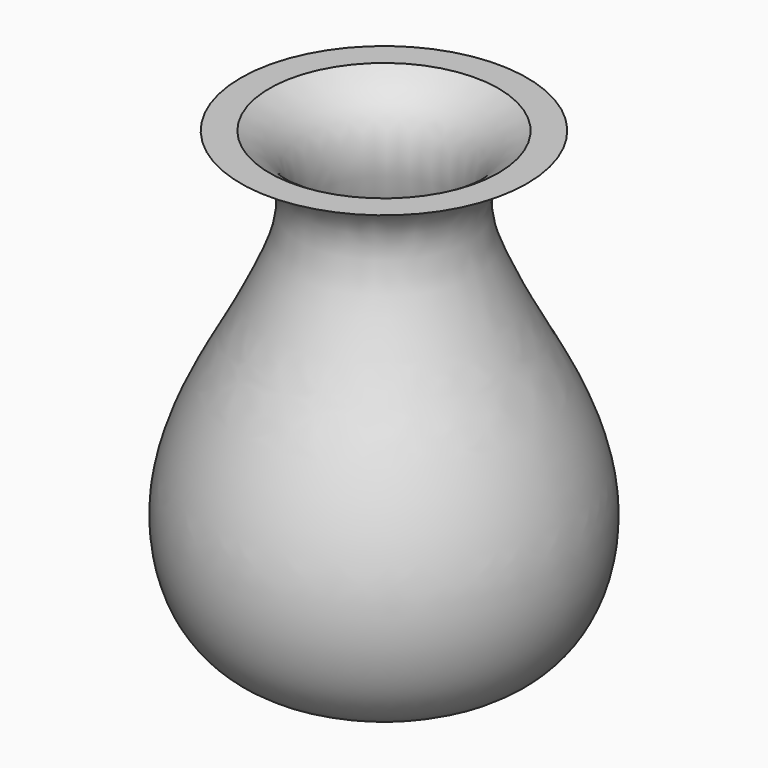
from build123d import *

# Parameters (mm, degrees)
F3_R     = 9.4302496374
F4_DEPTH = 6


# Not quite as in the source:
# - ends of sketch curves that miss each other by under 0.0002 mm in the source are joined
# - the dataset's text gives a spline's control points without its knots; the knots are read off the source's solid


with BuildPart() as f1:
    # F0 (on Front) → F1 (revolve)
    with BuildSketch(Plane.XZ):
        with BuildLine():
            add(Edge.make_bspline(
                [(30, 75.2996280789), (12.0761917662, 69.9585662546), (22.0660075591, 46.676498365), (27.6966733214, 36.2218981282), (42.7063983627, 9.1057052867), (34.5811633648, -19.2495821704), (17.7899881188, -23.4487943823), (14.7886006228, -24.1117397402)],
                knots=[0, 0, 0, 0, 0.1815872534, 0.3121168672, 0.4958376177, 0.6870531162, 0.7613433038, 0.7613433038, 0.7613433038, 0.7613433038], degree=3))
            Line((30, 75.2996280789), (23.9999937812, 75.2996280789))
            add(Edge.make_bspline(
                [(23.9999937812, 75.2996280789), (23.0401652673, 74.7936187135), (21.0247588483, 73.5335074467), (18.5585291762, 71.2374375612), (16.7198379267, 68.4175594433), (15.6826696477, 65.4130506141), (15.331612914, 62.3713239622), (15.5126860744, 59.3815893599), (16.0825011592, 56.4910760238), (16.916705774, 53.735455434), (17.7387201772, 51.5831610633), (18.4189479706, 49.9704141376), (18.9272543321, 48.8216741349), (19.4200549077, 47.7419083495), (20.0398236053, 46.399710855), (20.761807686, 44.8611954438), (21.562965975, 43.197405411), (22.321250427, 41.6663703234), (23.3029927321, 39.7404596384), (24.2824625412, 37.8948692714), (25.343200206, 35.9421986679), (26.2036248268, 34.371647892), (27.1429247952, 32.659191045), (28.4652186968, 30.2061159952), (30.1973374203, 26.8366561034), (32.2218636423, 22.3857513618), (34.0118488472, 17.6106526585), (35.1592588041, 13.4348404718), (35.785448931, 10.0199360293), (36.1877986343, 6.5714727134), (36.2397252491, 2.1938313072), (35.5493802078, -2.9499350247), (34.0820339451, -7.7778609851), (32.2029522741, -11.3746917966), (30.3010280758, -13.9131417929), (28.6716145167, -15.6306743639), (27.1396783972, -16.8932037461), (25.803572558, -17.7950920184), (24.39420105, -18.619315045), (22.4500071463, -19.5323385504), (20.4021028111, -20.2844311556), (18.7807315029, -20.7948544502), (17.592772776, -21.134210518), (16.452031039, -21.4325127884), (15.3771894816, -21.6925038619), (14.5514142739, -21.8797412312), (13.9410981585, -22.0135668432), (13.5103701444, -22.1064333576), (13.1083048799, -22.192326543), (12.7361659904, -22.2718756926), (12.3945880535, -22.3458779112), (12.0829949511, -22.4154919187), (11.8460619557, -22.4713734196), (11.6659844883, -22.5167836099), (11.5334752407, -22.5521765476), (11.4001289551, -22.5904987487), (11.2601656039, -22.6346104606), (11.1030535346, -22.6906076905), (10.9416605144, -22.7575957417), (10.7728572344, -22.8425122924), (10.6167334994, -22.9333364829), (10.4180576805, -23.0719896525), (10.1623729849, -23.2989454947), (9.8981203684, -23.6304309896), (9.7130739302, -24.0099991802), (9.6451369281, -24.2229738932), (9.6219207987, -24.3173828521)],
                knots=[0.0193804615, 0.0193804615, 0.0193804615, 0.0193804615, 0.0313625372, 0.0470438057, 0.0627250743, 0.0784063429, 0.0940876115, 0.1097688801, 0.1254501486, 0.1411314172, 0.1568126858, 0.1646533201, 0.1724939544, 0.1803345887, 0.188175223, 0.2038564915, 0.2195377601, 0.2352190287, 0.2509002973, 0.2822628344, 0.297944103, 0.3136253716, 0.3293066402, 0.3449879088, 0.3763504459, 0.4077129831, 0.4390755202, 0.4704380574, 0.486119326, 0.5018005946, 0.5331631317, 0.5645256689, 0.595888206, 0.6272507432, 0.6429320118, 0.6586132804, 0.6742945489, 0.6821351832, 0.6899758175, 0.7056570861, 0.7213383547, 0.729178989, 0.7370196233, 0.7448602576, 0.7527008918, 0.7605415261, 0.7644618433, 0.7683821604, 0.7723024776, 0.7762227947, 0.7801431119, 0.784063429, 0.7879837462, 0.7899439047, 0.7919040633, 0.7938642219, 0.7958243804, 0.797784539, 0.7997446976, 0.8007247769, 0.8017048562, 0.8026849354, 0.8036650147, 0.804645094, 0.8051351337, 0.8054861615, 0.8054861615, 0.8054861615, 0.8054861615], degree=3))
            Line((9.6219207987, -24.3173828521), (14.7886006228, -24.1117397402))
        make_face()
    revolve(axis=Axis((0, 0, 25.2996280789), (0, 0, -1)))


with BuildPart() as f1b:
    # F0 (on Front) → F1, piece 2 (revolve)
    with BuildSketch(Plane.XZ):
        with BuildLine():
            add(Edge.make_bspline(
                [(23.9999937812, 75.2996399804), (23.0401652673, 74.7936187135), (21.0247588483, 73.5335074467), (18.5585291762, 71.2374375612), (16.7198379267, 68.4175594433), (15.6826696477, 65.4130506141), (15.331612914, 62.3713239622), (15.5126860744, 59.3815893599), (16.0825011592, 56.4910760238), (16.916705774, 53.735455434), (17.7387201772, 51.5831610633), (18.4189479706, 49.9704141376), (18.9272543321, 48.8216741349), (19.4200549077, 47.7419083495), (20.0398236053, 46.399710855), (20.761807686, 44.8611954438), (21.562965975, 43.197405411), (22.321250427, 41.6663703234), (23.3029927321, 39.7404596384), (24.2824625412, 37.8948692714), (25.343200206, 35.9421986679), (26.2036248268, 34.371647892), (27.1429247952, 32.659191045), (28.4652186968, 30.2061159952), (30.1973374203, 26.8366561034), (32.2218636423, 22.3857513618), (34.0118488472, 17.6106526585), (35.1592588041, 13.4348404718), (35.785448931, 10.0199360293), (36.1877986343, 6.5714727134), (36.2397252491, 2.1938313072), (35.5493802078, -2.9499350247), (34.0820339451, -7.7778609851), (32.2029522741, -11.3746917966), (30.3010280758, -13.9131417929), (28.6716145167, -15.6306743639), (27.1396783972, -16.8932037461), (25.803572558, -17.7950920184), (24.39420105, -18.619315045), (22.4500071463, -19.5323385504), (20.4021028111, -20.2844311556), (18.7807315029, -20.7948544502), (17.592772776, -21.134210518), (16.452031039, -21.4325127884), (15.3771894816, -21.6925038619), (14.5514142739, -21.8797412312), (13.9410981585, -22.0135668432), (13.5103701444, -22.1064333576), (13.1083048799, -22.192326543), (12.7361659904, -22.2718756926), (12.3945880535, -22.3458779112), (12.0829949511, -22.4154919187), (11.8460619557, -22.4713734196), (11.6659844883, -22.5167836099), (11.5334752407, -22.5521765476), (11.4001289551, -22.5904987487), (11.2601656039, -22.6346104606), (11.1030535346, -22.6906076905), (10.9416605144, -22.7575957417), (10.7728572344, -22.8425122924), (10.6167334994, -22.9333364829), (10.4180576805, -23.0719896525), (10.1623729849, -23.2989454947), (9.8981203684, -23.6304309896), (9.7130739302, -24.0099991802), (9.6451369281, -24.2229738932), (9.6219207987, -24.3173828521)],
                knots=[0.0193804615, 0.0193804615, 0.0193804615, 0.0193804615, 0.0313625372, 0.0470438057, 0.0627250743, 0.0784063429, 0.0940876115, 0.1097688801, 0.1254501486, 0.1411314172, 0.1568126858, 0.1646533201, 0.1724939544, 0.1803345887, 0.188175223, 0.2038564915, 0.2195377601, 0.2352190287, 0.2509002973, 0.2822628344, 0.297944103, 0.3136253716, 0.3293066402, 0.3449879088, 0.3763504459, 0.4077129831, 0.4390755202, 0.4704380574, 0.486119326, 0.5018005946, 0.5331631317, 0.5645256689, 0.595888206, 0.6272507432, 0.6429320118, 0.6586132804, 0.6742945489, 0.6821351832, 0.6899758175, 0.7056570861, 0.7213383547, 0.729178989, 0.7370196233, 0.7448602576, 0.7527008918, 0.7605415261, 0.7644618433, 0.7683821604, 0.7723024776, 0.7762227947, 0.7801431119, 0.784063429, 0.7879837462, 0.7899439047, 0.7919040633, 0.7938642219, 0.7958243804, 0.797784539, 0.7997446976, 0.8007247769, 0.8017048562, 0.8026849354, 0.8036650147, 0.804645094, 0.8051351337, 0.8054861615, 0.8054861615, 0.8054861615, 0.8054861615], degree=3))
            Line((23.9999937812, 75.2996399804), (0, 75.2996280789))
            Line((0, 75.2996280789), (0, -24.7003719211))
            Line((0, -24.7003719211), (9.6219207987, -24.3173828521))
        make_face()
    revolve(axis=Axis((0, 0, 25.2996280789), (0, 0, -1)))

    # F0 (on Front) → F2 (revolve, cut)
    with BuildSketch(Plane.XZ):
        with BuildLine():
            add(Edge.make_bspline(
                [(23.9999937812, 75.2996399804), (23.0401652673, 74.7936187135), (21.0247588483, 73.5335074467), (18.5585291762, 71.2374375612), (16.7198379267, 68.4175594433), (15.6826696477, 65.4130506141), (15.331612914, 62.3713239622), (15.5126860744, 59.3815893599), (16.0825011592, 56.4910760238), (16.916705774, 53.735455434), (17.7387201772, 51.5831610633), (18.4189479706, 49.9704141376), (18.9272543321, 48.8216741349), (19.4200549077, 47.7419083495), (20.0398236053, 46.399710855), (20.761807686, 44.8611954438), (21.562965975, 43.197405411), (22.321250427, 41.6663703234), (23.3029927321, 39.7404596384), (24.2824625412, 37.8948692714), (25.343200206, 35.9421986679), (26.2036248268, 34.371647892), (27.1429247952, 32.659191045), (28.4652186968, 30.2061159952), (30.1973374203, 26.8366561034), (32.2218636423, 22.3857513618), (34.0118488472, 17.6106526585), (35.1592588041, 13.4348404718), (35.785448931, 10.0199360293), (36.1877986343, 6.5714727134), (36.2397252491, 2.1938313072), (35.5493802078, -2.9499350247), (34.0820339451, -7.7778609851), (32.2029522741, -11.3746917966), (30.3010280758, -13.9131417929), (28.6716145167, -15.6306743639), (27.1396783972, -16.8932037461), (25.803572558, -17.7950920184), (24.39420105, -18.619315045), (22.4500071463, -19.5323385504), (20.4021028111, -20.2844311556), (18.7807315029, -20.7948544502), (17.592772776, -21.134210518), (16.452031039, -21.4325127884), (15.3771894816, -21.6925038619), (14.5514142739, -21.8797412312), (13.9410981585, -22.0135668432), (13.5103701444, -22.1064333576), (13.1083048799, -22.192326543), (12.7361659904, -22.2718756926), (12.3945880535, -22.3458779112), (12.0829949511, -22.4154919187), (11.8460619557, -22.4713734196), (11.6659844883, -22.5167836099), (11.5334752407, -22.5521765476), (11.4001289551, -22.5904987487), (11.2601656039, -22.6346104606), (11.1030535346, -22.6906076905), (10.9416605144, -22.7575957417), (10.7728572344, -22.8425122924), (10.6167334994, -22.9333364829), (10.4180576805, -23.0719896525), (10.1623729849, -23.2989454947), (9.8981203684, -23.6304309896), (9.7130739302, -24.0099991802), (9.6451369281, -24.2229738932), (9.6219207987, -24.3173828521)],
                knots=[0.0193804615, 0.0193804615, 0.0193804615, 0.0193804615, 0.0313625372, 0.0470438057, 0.0627250743, 0.0784063429, 0.0940876115, 0.1097688801, 0.1254501486, 0.1411314172, 0.1568126858, 0.1646533201, 0.1724939544, 0.1803345887, 0.188175223, 0.2038564915, 0.2195377601, 0.2352190287, 0.2509002973, 0.2822628344, 0.297944103, 0.3136253716, 0.3293066402, 0.3449879088, 0.3763504459, 0.4077129831, 0.4390755202, 0.4704380574, 0.486119326, 0.5018005946, 0.5331631317, 0.5645256689, 0.595888206, 0.6272507432, 0.6429320118, 0.6586132804, 0.6742945489, 0.6821351832, 0.6899758175, 0.7056570861, 0.7213383547, 0.729178989, 0.7370196233, 0.7448602576, 0.7527008918, 0.7605415261, 0.7644618433, 0.7683821604, 0.7723024776, 0.7762227947, 0.7801431119, 0.784063429, 0.7879837462, 0.7899439047, 0.7919040633, 0.7938642219, 0.7958243804, 0.797784539, 0.7997446976, 0.8007247769, 0.8017048562, 0.8026849354, 0.8036650147, 0.804645094, 0.8051351337, 0.8054861615, 0.8054861615, 0.8054861615, 0.8054861615], degree=3))
            Line((23.9999937812, 75.2996399804), (0, 75.2996280789))
            Line((0, 75.2996280789), (0, -24.7003719211))
            Line((0, -24.7003719211), (9.6219207987, -24.3173828521))
        make_face()
    revolve(axis=Axis((0, 0, 25.2996280789), (0, 0, -1)), mode=Mode.SUBTRACT)


with BuildPart() as f4:
    # F3 (on Top) → F4 (new body)
    with BuildSketch(Plane.XY):
        Circle(F3_R)
    extrude(amount=F4_DEPTH)


solid = Compound([f1.part, f4.part])
